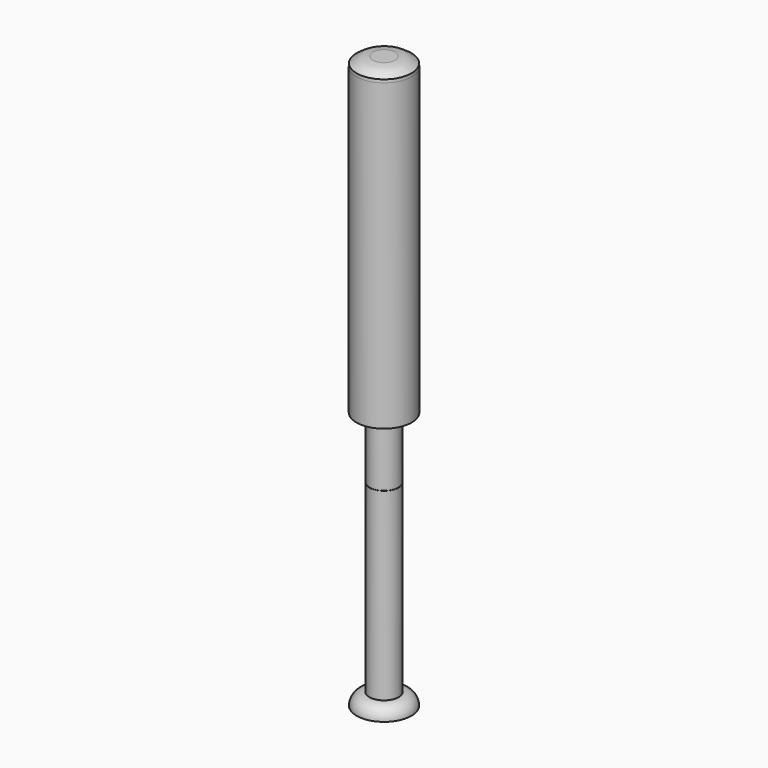
from build123d import *

# Parameters (mm, degrees)
F0_R      = 5.6573529482
F1_DEPTH  = 2.54
F2_R      = 2.53999
F3_R      = 3.0182712291
F4_DEPTH  = 38.1
F5_R      = 2.9745722731
F6_DEPTH  = 12.7
F7_R      = 5.6947098188
F7_R_2    = 2.9745722731
F8_DEPTH  = 63.5
F10_R     = 5.6566477781
F11_DEPTH = 1.27


# Not quite as in the source:
# - a fillet or chamfer that OpenCascade refuses, or shapes differently, is made with other operations: its cross-section is extruded or revolved along the edge and cut away or added
# - a fillet or chamfer is up to 0.001 mm smaller than in the source, because OpenCascade refuses the exact size
# - the program builds the solid bodies; features that only make, move or delete a surface that nothing else refers to are left out


with BuildPart() as f1:
    # F0 (on Top) → F1 (new body)
    with BuildSketch(Plane.XY):
        with Locations((-59.8805323243, -50.4733622074)):
            Circle(F0_R)
    extrude(amount=F1_DEPTH)

    # F2 (radius 2.54 in the source; OpenCascade refuses exactly that, so slightly less here)
    f2_edges = [f1.edges().sort_by_distance(p)[0] for p in [
        (-65.537885, -50.473362, 2.54),
    ]]
    fillet(f2_edges, radius=F2_R)

    # F3 (on face) → F4 (join)
    with BuildSketch(Plane.XY.offset(2.54)):
        with Locations((-59.8805323243, -50.4733622074)):
            Circle(F3_R)
    extrude(amount=F4_DEPTH)

    # F5 (on face) → F6 (join)
    with BuildSketch(Plane.XY.offset(40.64)):
        with Locations((-59.8805323243, -50.4733622074)):
            Circle(F5_R)
    extrude(amount=F6_DEPTH)


with BuildPart() as f8:
    # F7 (on face) → F8 (new body)
    with BuildSketch(Plane.XY.offset(53.34)):
        with Locations((-59.8805323243, -50.4733622074)):
            Circle(F7_R)
        with Locations((-59.8805323243, -50.4733622074)):
            Circle(F7_R_2, mode=Mode.SUBTRACT)
    extrude(amount=F8_DEPTH)

    # F10 (on face) → F11 (join)
    with BuildSketch(Plane.XY.offset(116.84)):
        with Locations((-59.8805323243, -50.4733622074)):
            Circle(F10_R)
    extrude(amount=F11_DEPTH)

    # F12: fillet of radius 5.08 on 2 edges, made by hand

    # F12_s1 → F12_t2 (revolve, cut)
    with BuildSketch(Plane.XZ.offset(50.4733622074)):
        with BuildLine():
            ThreePointArc((-54.2238845462, 116.84), (-55.7879374871, 117.7819048812), (-57.5839887113, 118.11))
            Line((-57.5839887113, 118.11), (-54.2238845462, 118.11))
            Line((-54.2238845462, 118.11), (-54.2238845462, 116.84))
        make_face()
    revolve(axis=Axis((-59.8805323243, -50.4733622074, 118.11), (0, 0, 1)), mode=Mode.SUBTRACT)

    # F12_s3 → F12_t4 (revolve, cut)
    with BuildSketch(Plane.XZ.offset(50.4733622074)):
        with BuildLine():
            ThreePointArc((-54.1858225055, 116.2193055383), (-54.1953469443, 116.5302357289), (-54.2238845462, 116.84))
            Line((-54.2238845462, 116.84), (-54.1858225055, 116.84))
            Line((-54.1858225055, 116.84), (-54.1858225055, 116.2193055383))
        make_face()
    revolve(axis=Axis((-59.8805323243, -50.4733622074, 116.84), (0, 0, 1)), mode=Mode.SUBTRACT)


solid = Compound([f1.part, f8.part])
